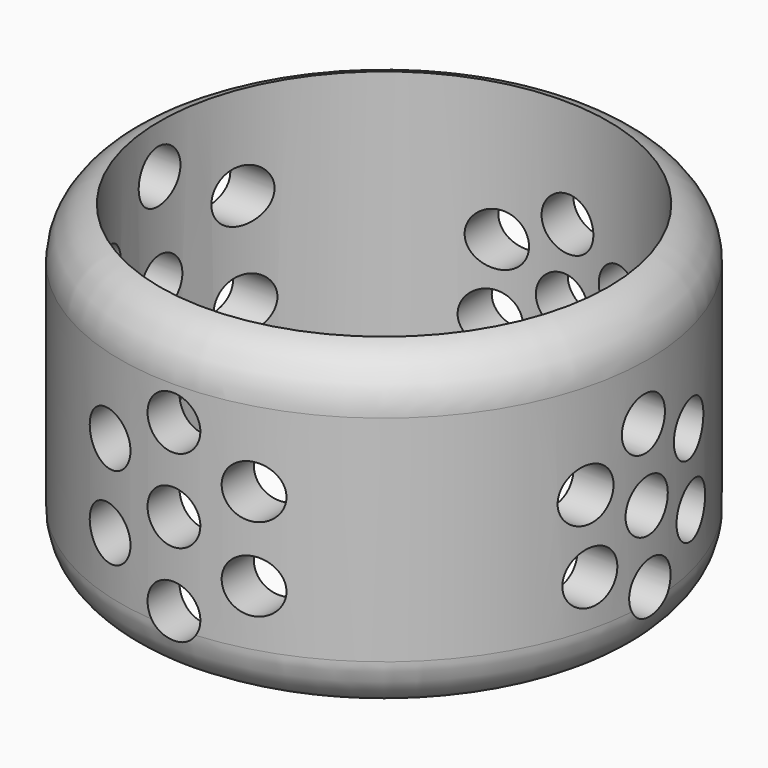
from build123d import *

# Parameters (mm, degrees)
F0_R      = 10
F0_R_2    = 8.5
F1_DEPTH  = 12
F4_D      = 2
F4_DEPTH  = 10.001
F6_D      = 2
F6_DEPTH  = 10.0010001
F8_D      = 2
F8_DEPTH  = 10.0010001
F10_D     = 2
F10_DEPTH = 10.0010001


# Not quite as in the source:
# - a fillet or chamfer that OpenCascade refuses, or shapes differently, is made with other operations: its cross-section is extruded or revolved along the edge and cut away or added


with BuildPart() as f1:
    # F0 (on Top) → F1 (new body)
    with BuildSketch(Plane.XY):
        Circle(F0_R)
        Circle(F0_R_2, mode=Mode.SUBTRACT)
    extrude(amount=F1_DEPTH)

    # F2: fillet of radius 2 on 2 edges, made by hand

    # F2_s1 → F2_t2 (revolve, cut)
    with BuildSketch(Plane.XZ):
        with BuildLine():
            ThreePointArc((10, 10.0635083269), (9.5811388301, 11.2882531983), (8.5, 12))
            Line((8.5, 12), (10, 12))
            Line((10, 12), (10, 10.0635083269))
        make_face()
    revolve(axis=Axis((0, 0, 12), (0, 0, 1)), mode=Mode.SUBTRACT)

    # F2_s3 → F2_t4 (revolve, cut)
    with BuildSketch(Plane.XZ):
        with BuildLine():
            ThreePointArc((10, 1.9364916731), (9.5811388301, 0.7117468017), (8.5, 0))
            Line((8.5, 0), (10, 0))
            Line((10, 0), (10, 1.9364916731))
        make_face()
    revolve(axis=Axis((0, 0, 0), (0, 0, 1)), mode=Mode.SUBTRACT)

    # F4 (through all, one way)
    with BuildSketch(Plane(origin=(0, 0, 0), x_dir=(1, 0, 0), z_dir=(0, 1, 0))):
        with Locations((0, -8.780693493), (2.7273921296, -7.2060329128), (2.7273921296, -4.0567117524), (0, -2.4820511722), (-2.7273921296, -4.0567117524), (-2.7273921296, -7.2060329128), (0, -5.6313723326)):
            Circle(F4_D / 2)
    extrude(amount=-F4_DEPTH, mode=Mode.SUBTRACT)

    # F6 (through all, one way)
    with BuildSketch(Plane(origin=(0, 0, 0), x_dir=(0, 1, 0), z_dir=(-1, 0, 0))):
        with Locations((-0.1533140905, -7.9868231674), (2.3390492435, -6.7248883884), (2.492363334, -3.9354710361), (0.1533140905, -2.4079884629), (-2.3390492435, -3.6699232419), (-2.492363334, -6.4593405941), (0, -5.1974058151)):
            Circle(F6_D / 2)
    extrude(amount=-F6_DEPTH, mode=Mode.SUBTRACT)

    # F8 (through all, one way)
    with BuildSketch(Plane.XZ):
        with Locations((0.1981962625, 7.9384916561), (0, 5.2428534254), (2.4335893184, 6.4190295426), (2.235393056, 3.7233913119), (-0.1981962625, 2.5472151948), (-2.4335893184, 4.0666773083), (-2.235393056, 6.762315539)):
            Circle(F8_D / 2)
    extrude(amount=-F8_DEPTH, mode=Mode.SUBTRACT)

    # F10 (through all, one way)
    with BuildSketch(Plane.YZ):
        with Locations((-0.0803171602, 10.1880325247), (0, 6.5471483395), (3.1129396166, 8.4371471331), (3.1932567767, 4.7962629479), (-3.1129396166, 4.6571495458), (-3.1932567767, 8.298033731), (0.0803171602, 2.9062641542)):
            Circle(F10_D / 2)
    extrude(amount=-F10_DEPTH, mode=Mode.SUBTRACT)


solid = f1.part
